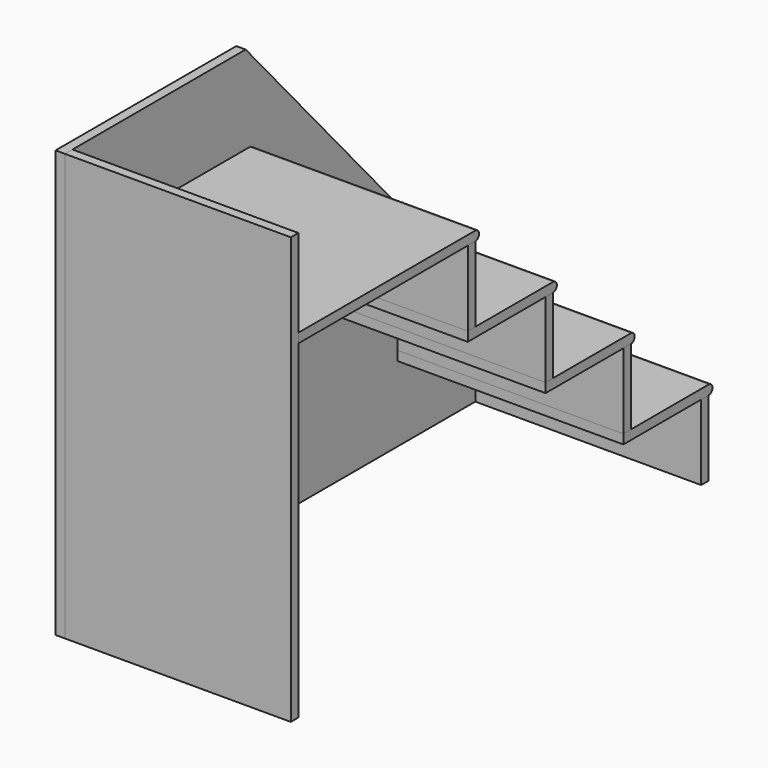
from build123d import *

# Parameters (mm, degrees)
F1_DEPTH = 19.05
F2_W     = 19.05
F2_H     = 863.6
F3_DEPTH = 457.2
F4_W     = 457.2
F4_H     = 19.05
F5_DEPTH = 457.2
F4_W_2   = 225.425
F6_R     = 9.52499
F6_2_R   = 9.52499
F6_3_R   = 9.52499
F6_4_R   = 9.52499
F7_W     = 19.05
F7_H     = 152.4
F8_DEPTH = 457.2


# Not quite as in the source:
# - a fillet or chamfer is up to 0.001 mm smaller than in the source, because OpenCascade refuses the exact size


with BuildPart() as f1:
    # F0 (on Right) → F1 (new body)
    with BuildSketch(Plane.YZ):
        Polygon((-609.6, 863.6), (-1066.8, 863.6), (-1066.8, 0), (0, 0), (0, 177.8), align=None)
    extrude(amount=F1_DEPTH)


with BuildPart() as f3:
    # F2 (on face) → F3 (new body)
    with BuildSketch(Plane.YZ.offset(19.05)):
        with Locations((-1057.275, 431.8)):
            Rectangle(F2_W, F2_H)
    extrude(amount=F3_DEPTH)


with BuildPart() as f5:
    # F4 (on face) → F5 (new body, through all)
    with BuildSketch(Plane.YZ.offset(19.05)):
        with Locations((-819.15, 676.275)):
            Rectangle(F4_W, F4_H)
    extrude(amount=F5_DEPTH)

    # F6 (radius 9.525 in the source; OpenCascade refuses exactly that, so slightly less here)
    f6_edges = [f5.edges().sort_by_distance(p)[0] for p in [
        (247.65, -590.55, 685.8),
        (247.65, -590.55, 666.75),
    ]]
    fillet(f6_edges, radius=F6_R)


with BuildPart() as f5b:
    # F4 (on face) → F5, piece 2 (new body, through all)
    with BuildSketch(Plane.YZ.offset(19.05)):
        with Locations((-112.7125, 161.925)):
            Rectangle(F4_W_2, F4_H)
    extrude(amount=F5_DEPTH)

    # F6#4 (radius 9.525 in the source; OpenCascade refuses exactly that, so slightly less here)
    f6_4_edges = [f5b.edges().sort_by_distance(p)[0] for p in [
        (247.65, 0, 171.45),
        (247.65, 0, 152.4),
    ]]
    fillet(f6_4_edges, radius=F6_4_R)


with BuildPart() as f5c:
    # F4 (on face) → F5, piece 3 (new body, through all)
    with BuildSketch(Plane.YZ.offset(19.05)):
        with Locations((-309.5625, 333.375)):
            Rectangle(F4_W_2, F4_H)
    extrude(amount=F5_DEPTH)

    # F6#3 (radius 9.525 in the source; OpenCascade refuses exactly that, so slightly less here)
    f6_3_edges = [f5c.edges().sort_by_distance(p)[0] for p in [
        (247.65, -196.85, 342.9),
        (247.65, -196.85, 323.85),
    ]]
    fillet(f6_3_edges, radius=F6_3_R)


with BuildPart() as f5d:
    # F4 (on face) → F5, piece 4 (new body, through all)
    with BuildSketch(Plane.YZ.offset(19.05)):
        with Locations((-506.4125, 504.825)):
            Rectangle(F4_W_2, F4_H)
    extrude(amount=F5_DEPTH)

    # F6#2 (radius 9.525 in the source; OpenCascade refuses exactly that, so slightly less here)
    f6_2_edges = [f5d.edges().sort_by_distance(p)[0] for p in [
        (247.65, -393.7, 514.35),
        (247.65, -393.7, 495.3),
    ]]
    fillet(f6_2_edges, radius=F6_2_R)


with BuildPart() as f8:
    # F7 (on face) → F8 (new body, through all)
    with BuildSketch(Plane.YZ.offset(19.05)):
        with Locations((-609.6, 590.55)):
            Rectangle(F7_W, F7_H)
    extrude(amount=F8_DEPTH)


with BuildPart() as f8b:
    # F7 (on face) → F8, piece 2 (new body, through all)
    with BuildSketch(Plane.YZ.offset(19.05)):
        with Locations((-412.75, 419.1)):
            Rectangle(F7_W, F7_H)
    extrude(amount=F8_DEPTH)


with BuildPart() as f8c:
    # F7 (on face) → F8, piece 3 (new body, through all)
    with BuildSketch(Plane.YZ.offset(19.05)):
        with Locations((-215.9, 247.65)):
            Rectangle(F7_W, F7_H)
    extrude(amount=F8_DEPTH)


with BuildPart() as f8d:
    # F7 (on face) → F8, piece 4 (new body, through all)
    with BuildSketch(Plane.YZ.offset(19.05)):
        with Locations((-19.05, 76.2)):
            Rectangle(F7_W, F7_H)
    extrude(amount=F8_DEPTH)


solid = Compound([f1.part, f3.part, f5.part, f5b.part, f5c.part, f5d.part, f8.part, f8b.part, f8c.part, f8d.part])
